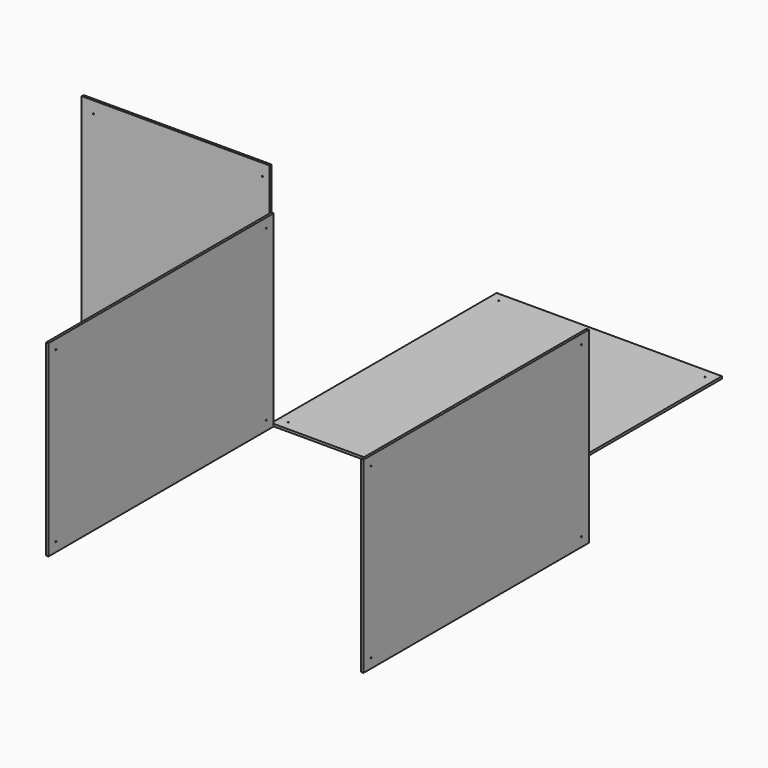
from build123d import *

# Parameters (mm, degrees)
F1_W     = 609.6
F1_H     = 762
F1_R     = 1.5875
F3_DEPTH = 6.35
F5_W     = 762
F5_H     = 508
F5_R     = 1.5875
F6_DEPTH = 6.35
F8_W     = 508
F8_H     = 622.3
F8_R     = 1.5875
F9_DEPTH = 6.35


# Not quite as in the source:
# - a variable given as a bare number and used for a length is read in inches; the dataset says mm whatever the document's units were


with BuildPart() as f3:
    # F1 (on face) → F3 (new body)
    with BuildSketch(Plane.XY):
        with Locations((304.8, 381)):
            Rectangle(F1_W, F1_H)
        with Locations((25.4, 25.4)):
            Circle(F1_R, mode=Mode.SUBTRACT)
        with Locations((584.2, 25.4)):
            Circle(F1_R, mode=Mode.SUBTRACT)
        with Locations((25.4, 736.6)):
            Circle(F1_R, mode=Mode.SUBTRACT)
        with Locations((584.2, 736.6)):
            Circle(F1_R, mode=Mode.SUBTRACT)
    extrude(amount=F3_DEPTH)


with BuildPart() as f6:
    # F5 (on face) → F6 (new body)
    with BuildSketch(Plane.YZ):
        with Locations((-381, 254)):
            Rectangle(F5_W, F5_H)
        with Locations((-736.6, 25.4)):
            Circle(F5_R, mode=Mode.SUBTRACT)
        with Locations((-25.4, 25.4)):
            Circle(F5_R, mode=Mode.SUBTRACT)
        with Locations((-736.6, 482.6)):
            Circle(F5_R, mode=Mode.SUBTRACT)
        with Locations((-25.4, 482.6)):
            Circle(F5_R, mode=Mode.SUBTRACT)
    extrude(amount=F6_DEPTH)


with BuildPart() as f7_1:
    # F7: copy of F6
    add(f6.part.moved(Location((852.68034, 0, 0))))


with BuildPart() as f9:
    # F8 (on Front) → F9 (new body)
    with BuildSketch(Plane.XZ):
        with Locations((-254, 311.15)):
            Rectangle(F8_W, F8_H)
        with Locations((-476.25, 31.75)):
            Circle(F8_R, mode=Mode.SUBTRACT)
        with Locations((-19.05, 31.75)):
            Circle(F8_R, mode=Mode.SUBTRACT)
        with Locations((-476.25, 590.55)):
            Circle(F8_R, mode=Mode.SUBTRACT)
        with Locations((-19.05, 590.55)):
            Circle(F8_R, mode=Mode.SUBTRACT)
    extrude(amount=F9_DEPTH)


solid = Compound([f3.part, f6.part, f7_1.part, f9.part])
